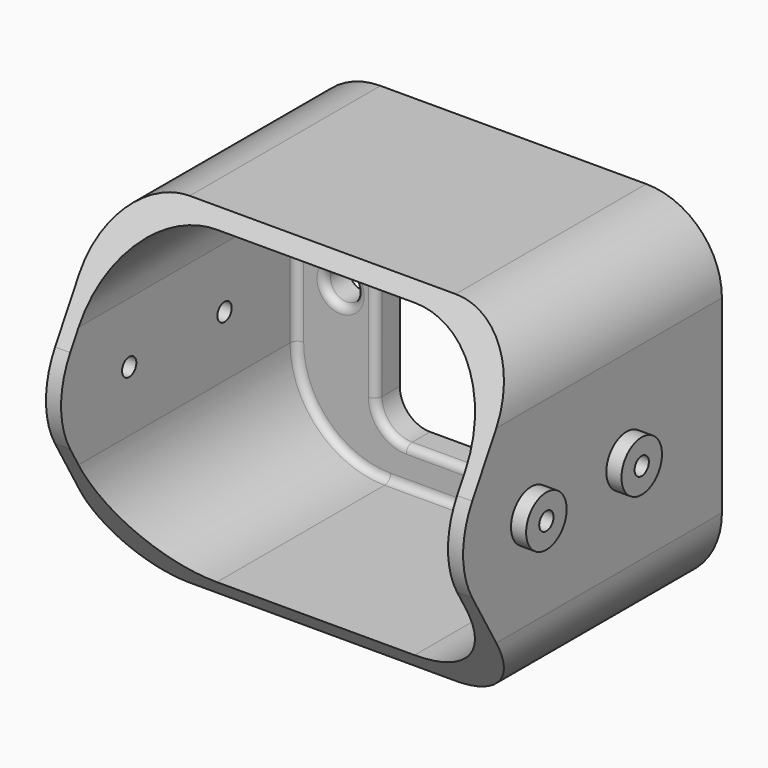
from build123d import *
from build123d import SkipClean  # not in build123d's __all__

# Parameters (mm, degrees)
F0_R           = 1.0795
F1_DEPTH       = 2
F3_DEPTH       = 19.9898
F4_R           = 0.508
F5_R           = 0.6
F6_DEPTH       = 28.0045
F7_R           = 1.7
F7_R_2         = 0.6
F8_DEPTH       = 1.016
F9_R           = 1.7
F9_R_2         = 0.6
F10_DEPTH      = 1.016
F12_DEPTH      = 15.01875
F12_DEPTH_BACK = 15.01875


# Not quite as in the source:
# - after a boolean that leaves OpenCascade's solid faulty, fix() repairs it


with BuildPart() as f1:
    # F0 (on Front) → F1 (new body)
    with BuildSketch(Plane.XZ):
        with BuildLine():
            Line((8.92175, 11.43), (-8.92175, 11.43))
            ThreePointArc((-8.92175, 11.43), (-12.5138524484, 9.9421024484), (-14.00175, 6.35))
            Line((-14.00175, 6.35), (-14.00175, -6.35))
            ThreePointArc((-14.00175, -6.35), (-12.5138524484, -9.9421024484), (-8.92175, -11.43))
            Line((-8.92175, -11.43), (8.92175, -11.43))
            ThreePointArc((8.92175, -11.43), (12.5138524484, -9.9421024484), (14.00175, -6.35))
            Line((14.00175, -6.35), (14.00175, 6.35))
            ThreePointArc((14.00175, 6.35), (12.5138524484, 9.9421024484), (8.92175, 11.43))
        make_face()
        with Locations((-9.9949, 0)):
            Circle(F0_R, mode=Mode.SUBTRACT)
        with BuildLine():
            ThreePointArc((-7.62, 5.9055), (-7.0248409794, 7.3423409794), (-5.588, 7.9375))
            Line((-5.588, 7.9375), (5.588, 7.9375))
            ThreePointArc((5.588, 7.9375), (7.0248409794, 7.3423409794), (7.62, 5.9055))
            Line((7.62, 5.9055), (7.62, -5.9055))
            ThreePointArc((7.62, -5.9055), (7.0248409794, -7.3423409794), (5.588, -7.9375))
            Line((5.588, -7.9375), (-5.588, -7.9375))
            ThreePointArc((-5.588, -7.9375), (-7.0248409794, -7.3423409794), (-7.62, -5.9055))
            Line((-7.62, -5.9055), (-7.62, 5.9055))
        make_face(mode=Mode.SUBTRACT)
        with Locations((9.9949, 0)):
            Circle(F0_R, mode=Mode.SUBTRACT)
    extrude(amount=F1_DEPTH)

    # F2 (on face) → F3 (join)
    with BuildSketch(Plane.XZ.offset(2)):
        with BuildLine():
            Line((8.92175, 11.43), (-8.92175, 11.43))
            ThreePointArc((-8.92175, 11.43), (-12.5138524484, 9.9421024484), (-14.00175, 6.35))
            Line((-14.00175, 6.35), (-14.00175, -6.35))
            ThreePointArc((-14.00175, -6.35), (-12.5138524484, -9.9421024484), (-8.92175, -11.43))
            Line((-8.92175, -11.43), (8.92175, -11.43))
            ThreePointArc((8.92175, -11.43), (12.5138524484, -9.9421024484), (14.00175, -6.35))
            Line((14.00175, -6.35), (14.00175, 6.35))
            ThreePointArc((14.00175, 6.35), (12.5138524484, 9.9421024484), (8.92175, 11.43))
        make_face()
        with BuildLine():
            ThreePointArc((-12.98575, 4.064), (-11.1258780605, 8.5541280605), (-6.63575, 10.414))
            Line((-6.63575, 10.414), (6.63575, 10.414))
            ThreePointArc((6.63575, 10.414), (11.1258780605, 8.5541280605), (12.98575, 4.064))
            Line((12.98575, 4.064), (12.98575, -4.064))
            ThreePointArc((12.98575, -4.064), (11.1258780605, -8.5541280605), (6.63575, -10.414))
            Line((6.63575, -10.414), (-6.63575, -10.414))
            ThreePointArc((-6.63575, -10.414), (-11.1258780605, -8.5541280605), (-12.98575, -4.064))
            Line((-12.98575, -4.064), (-12.98575, 4.064))
        make_face(mode=Mode.SUBTRACT)
    extrude(amount=F3_DEPTH)

    # F4
    f4_edges = [f1.edges().sort_by_distance(p)[0] for p in [
        (-11.125878, -2, -8.554128),
        (-12.98575, -2, 0),
        (-11.125878, -2, 8.554128),
        (0, -2, 10.414),
        (11.125878, -2, 8.554128),
        (12.98575, -2, 0),
        (11.125878, -2, -8.554128),
        (0, -2, -10.414),
        (-11.0744, -2, 0),
        (-7.62, -2, 0),
        (-7.024841, -2, -7.342341),
        (-7.024841, -2, 7.342341),
        (0, -2, -7.9375),
        (0, -2, 7.9375),
        (7.024841, -2, -7.342341),
        (7.024841, -2, 7.342341),
        (7.62, -2, 0),
        (8.9154, -2, 0),
    ]]
    fillet(f4_edges, radius=F4_R)

    # F5 (on face) → F6 (cut, through all)
    with BuildSketch(Plane.YZ.offset(14.00175)):
        with Locations((-8, 0)):
            Circle(F5_R)
        with Locations((-16, 0)):
            Circle(F5_R)
    extrude(amount=-F6_DEPTH, mode=Mode.SUBTRACT)

    # F7 (on face) → F8 (join)
    with BuildSketch(Plane.YZ.offset(14.00175)):
        with Locations((-8, 0)):
            Circle(F7_R)
        with Locations((-8, 0)):
            Circle(F7_R_2, mode=Mode.SUBTRACT)
        with Locations((-16, 0)):
            Circle(F7_R)
        with Locations((-16, 0)):
            Circle(F7_R_2, mode=Mode.SUBTRACT)
    extrude(amount=F8_DEPTH)

    # F9 (on face) → F10 (join)
    with BuildSketch(Plane(origin=(-14.00175, 0, 0), x_dir=(0, -1, 0), z_dir=(-1, 0, 0))):
        with Locations((16, 0)):
            Circle(F9_R)
        with Locations((16, 0)):
            Circle(F9_R_2, mode=Mode.SUBTRACT)
        with Locations((8, 0)):
            Circle(F9_R)
        with Locations((8, 0)):
            Circle(F9_R_2, mode=Mode.SUBTRACT)
    with SkipClean():  # cleaning this boolean's faces spoils the solid; the shape is the same uncleaned
        extrude(amount=F10_DEPTH)

    # F11 (on Right) → F12 (cut, two sides)
    with BuildSketch(Plane.YZ) as f12_sk:
        with BuildLine():
            ThreePointArc((-20.9493351826, -2.8575), (-21.715, 0), (-20.9493351826, 2.8575))
            Line((-20.9493351826, 2.8575), (-14.935231149, 13.2742337482))
            Line((-14.935231149, 13.2742337482), (-27.6412566526, 12.4483415457))
            Line((-27.6412566526, 12.4483415457), (-27.6412566526, -22.2988429875))
            Line((-27.6412566526, -22.2988429875), (-9.7248705754, -22.2988429875))
            Line((-9.7248705754, -22.2988429875), (-20.9493351826, -2.8575))
        make_face()
    extrude(amount=-F12_DEPTH, mode=Mode.SUBTRACT)
    extrude(f12_sk.sketch, amount=F12_DEPTH_BACK, mode=Mode.SUBTRACT)

    add(f1.part.fix(), mode=Mode.REPLACE)


solid = f1.part
